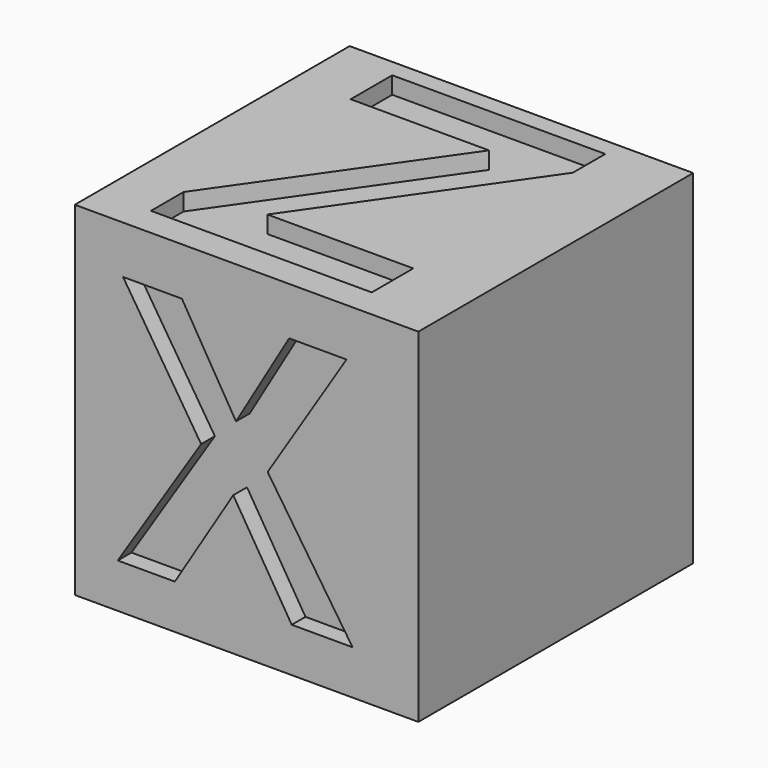
from build123d import *

# Parameters (mm, degrees)
F0_W         = 25.4
F0_H         = 25.4
F1_DEPTH     = 25.4
F2_TEXT_SIZE = 26.0290350128
F3_DEPTH     = 1.27
F4_TEXT_SIZE = 27.6525289181
F5_DEPTH     = 1.27
F6_TEXT_SIZE = 30.7258064516
F7_DEPTH     = 1.27


# Not quite as in the source:
# - Text() gives the source's letters only with a copy of the font that has no kerning and outlines rounded to 1/6400 em; it was checked with that copy


with BuildPart() as f1:
    # F0 (on Top) → F1 (new body)
    with BuildSketch(Plane.XY):
        Rectangle(F0_W, F0_H)
    extrude(amount=F1_DEPTH)

    # F2 (on face) → F3 (cut)
    with BuildSketch(Plane.XZ.offset(12.7)):
        with Locations((-9.525, 3.2780315969)):
            Text('X', F2_TEXT_SIZE, font='Open Sans', font_style=FontStyle.BOLD, text_align=(TextAlign.LEFT, TextAlign.BOTTOM))
    extrude(amount=-F3_DEPTH, mode=Mode.SUBTRACT)

    # F4 (on face) → F5 (cut)
    with BuildSketch(Plane(origin=(-12.7, 0, 0), x_dir=(0, -1, 0), z_dir=(-1, 0, 0))):
        with Locations((-9.525, 3.175)):
            Text('Y', F4_TEXT_SIZE, font='Open Sans', font_style=FontStyle.BOLD, text_align=(TextAlign.LEFT, TextAlign.BOTTOM))
    extrude(amount=-F5_DEPTH, mode=Mode.SUBTRACT)

    # F6 (on face) → F7 (cut)
    with BuildSketch(Plane.XY.offset(25.4)):
        with Locations((-9.525, -10.5491935484)):
            Text('Z', F6_TEXT_SIZE, font='Open Sans', font_style=FontStyle.BOLD, text_align=(TextAlign.LEFT, TextAlign.BOTTOM))
    extrude(amount=-F7_DEPTH, mode=Mode.SUBTRACT)


solid = f1.part
